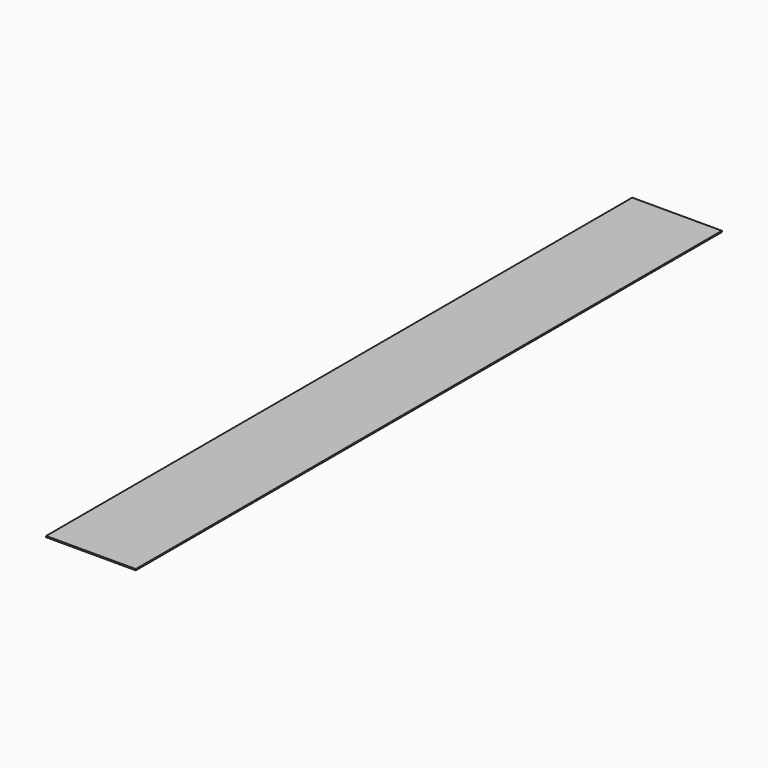
from build123d import *

# Parameters (mm, degrees)
F0_W     = 60
F0_H     = 490
F1_DEPTH = 0.79375


# Not quite as in the source:
# - a length typed as a fraction of an inch, garbled in the dataset ("3 / 203.2 mm" for 3/8 in), is restored


with BuildPart() as f1:
    # F0 (on Top) → F1 (new body)
    with BuildSketch(Plane.XY):
        Rectangle(F0_W, F0_H)
    extrude(amount=F1_DEPTH)


solid = f1.part
